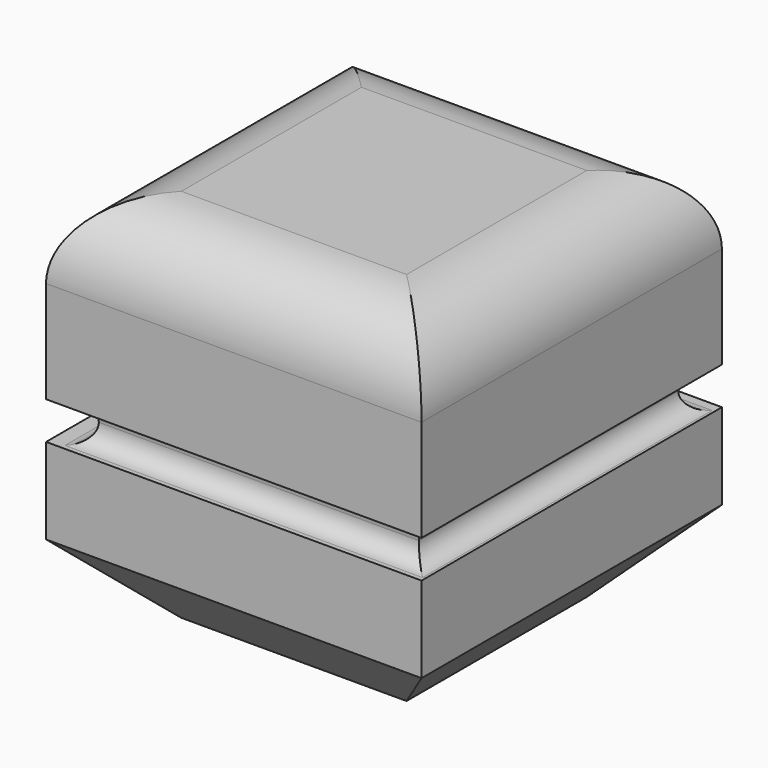
from build123d import *

# Parameters (mm, degrees)
F0_W     = 25.4
F0_H     = 25.4
F1_DEPTH = 25.4
F2_R     = 5.08
F3_SIZE  = 5.08
F4_W     = 25.741957128
F4_H     = 25.5791675299
F4_W_2   = 21.6466449201
F4_H_2   = 21.9391710125
F5_DEPTH = 2.54
F6_R     = 1.26999


# Not quite as in the source:
# - a fillet or chamfer is up to 0.001 mm smaller than in the source, because OpenCascade refuses the exact size


with BuildPart() as f1:
    # F0 (on Front) → F1 (new body)
    with BuildSketch(Plane.XZ):
        with Locations((-48.8445848724, -0.7304809988)):
            Rectangle(F0_W, F0_H)
    extrude(amount=F1_DEPTH)

    # F2
    f2_edges = [f1.edges().sort_by_distance(p)[0] for p in [
        (-48.844585, -25.4, 11.969519),
        (-36.144585, -12.7, 11.969519),
        (-48.844585, 0, 11.969519),
        (-61.544585, -12.7, 11.969519),
    ]]
    fillet(f2_edges, radius=F2_R)

    # F3
    f3_edges = [f1.edges().sort_by_distance(p)[0] for p in [
        (-48.844585, -25.4, -13.430481),
        (-36.144585, -12.7, -13.430481),
        (-61.544585, -12.7, -13.430481),
        (-48.844585, 0, -13.430481),
    ]]
    chamfer(f3_edges, length=F3_SIZE)

    # F4 (on Top) → F5 (cut)
    with BuildSketch(Plane.XY):
        with Locations((-48.707395792, -12.789583765)):
            Rectangle(F4_W, F4_H)
        with Locations((-48.4148729593, -12.8544487525)):
            Rectangle(F4_W_2, F4_H_2, mode=Mode.SUBTRACT)
    extrude(amount=-F5_DEPTH, mode=Mode.SUBTRACT)

    # F6 (radius 1.27 in the source; OpenCascade refuses exactly that, so slightly less here)
    f6_edges = [f1.edges().sort_by_distance(p)[0] for p in [
        (-48.414873, -1.884863, -2.54),
        (-37.59155, -12.854449, -2.54),
        (-48.414873, -1.884863, 0),
        (-37.59155, -12.854449, 0),
        (-48.414873, -23.824034, -2.54),
        (-59.238195, -12.854449, -2.54),
        (-48.414873, -23.824034, 0),
        (-59.238195, -12.854449, 0),
    ]]
    fillet(f6_edges, radius=F6_R)


solid = f1.part
